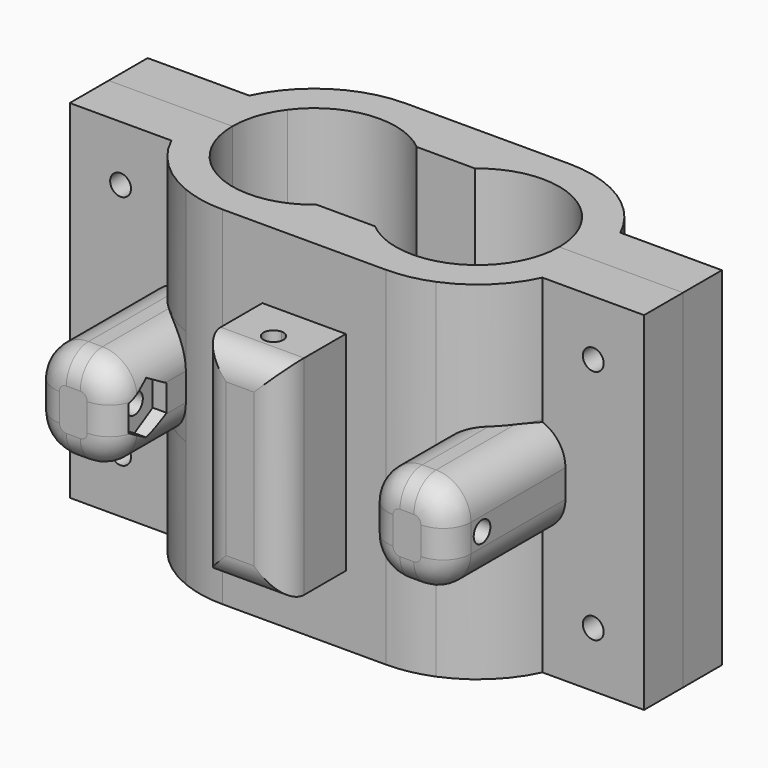
from build123d import *

# Parameters (mm, degrees)
F0_W           = 5.8084472025
F0_H           = 7
F0_W_2         = 1.5
F1_DEPTH       = 50
F2_DEPTH       = 50
F10_START      = -4
F10_DEPTH      = 21
F13_START      = 18
F13_DEPTH      = 14
F11_R          = 1.5
F14_DEPTH      = 35
F14_DEPTH_BACK = 35
F15_R          = 4
F16_START      = 10
F16_DEPTH      = 30
F17_R          = 4
F18_T2_ANGLE   = 90
F18_T4_ANGLE   = 90
F18_T6_ANGLE   = 90
F18_T8_ANGLE   = 90
F18_T10_ANGLE  = 90
F18_T12_ANGLE  = 90
F18_T14_ANGLE  = 90
F18_T16_ANGLE  = 90
F18_T20_DEPTH  = 21
F18_S21_R      = 16.5
F18_T22_DEPTH  = 13
F18_T26_DEPTH  = 21
F18_S27_R      = 16.5
F18_T28_DEPTH  = 13
F18_T32_DEPTH  = 25.2295219459
F18_S33_R      = 16.5
F18_T34_DEPTH  = 15
F18_T38_DEPTH  = 25.2295219459
F18_S39_R      = 16.5
F18_T40_DEPTH  = 15
F18_T44_DEPTH  = 25.2295219459
F18_S45_R      = 16.5
F18_T46_DEPTH  = 15
F18_T50_DEPTH  = 25.2295219459
F18_S51_R      = 16.5
F18_T52_DEPTH  = 15
F18_T56_DEPTH  = 21
F18_S57_R      = 16.5
F18_T58_DEPTH  = 13
F18_T62_DEPTH  = 21
F18_S63_R      = 16.5
F18_T64_DEPTH  = 13
F19_START      = -10
F19_DEPTH      = 10
F20_START      = 10
F20_DEPTH      = 10


# Not quite as in the source:
# - a fillet or chamfer that OpenCascade refuses, or shapes differently, is made with other operations: its cross-section is extruded or revolved along the edge and cut away or added
# - a feature names something its author has since deleted; it is built from what else it names


with BuildPart() as f1:
    # F0 (on Top) → F1 (new body)
    with BuildSketch(Plane.XY):
        with BuildLine():
            Line((-26.6915527975, 7), (-21.1872930441, 7))
            ThreePointArc((-21.1872930441, 7), (-13.1235807588, 11.6694376856), (-4.1960275351, 9))
            Line((-4.1960275351, 9), (4.1960275351, 9))
            ThreePointArc((4.1960275351, 9), (13.1235807588, 11.6694376856), (21.1872930441, 7))
            Line((21.1872930441, 7), (26.6915527975, 7))
            ThreePointArc((26.6915527975, 7), (20.6029656048, 13.9239003156), (11.75, 16.5))
            ThreePointArc((11.75, 16.5), (5.3815186987, 15.2214469061), (0, 11.5839328382))
            ThreePointArc((0, 11.5839328382), (-5.3815186987, 15.2214469061), (-11.75, 16.5))
            ThreePointArc((-11.75, 16.5), (-20.6029656048, 13.9239003156), (-26.6915527975, 7))
        make_face()
        with Locations((38.4042236013, 3.5)):
            Rectangle(F0_W, F0_H)
        with Locations((-38.4042236013, 3.5)):
            Rectangle(F0_W, F0_H)
        with Locations((-34.75, 3.5)):
            Rectangle(F0_W_2, F0_H)
        with Locations((-33.25, 3.5)):
            Rectangle(F0_W_2, F0_H)
        with BuildLine():
            Line((-32.5, 0), (-28.25, 0))
            ThreePointArc((-28.25, 0), (-27.8556763465, 3.585692321), (-26.6915527975, 7))
            Line((-26.6915527975, 7), (-32.5, 7))
            Line((-32.5, 7), (-32.5, 0))
        make_face()
        with Locations((33.25, 3.5)):
            Rectangle(F0_W_2, F0_H)
        with BuildLine():
            ThreePointArc((26.6915527975, 7), (27.8556763465, 3.585692321), (28.25, 0))
            Line((28.25, 0), (32.5, 0))
            Line((32.5, 0), (32.5, 7))
            Line((32.5, 7), (26.6915527975, 7))
        make_face()
        with Locations((34.75, 3.5)):
            Rectangle(F0_W_2, F0_H)
        with BuildLine():
            Line((-28.25, 0), (-23.5, 0))
            ThreePointArc((-23.5, 0), (-22.9068520038, 3.686075605), (-21.1872930441, 7))
            Line((-21.1872930441, 7), (-26.6915527975, 7))
            ThreePointArc((-26.6915527975, 7), (-27.8556763465, 3.585692321), (-28.25, 0))
        make_face()
        with BuildLine():
            ThreePointArc((21.1872930441, 7), (22.9068520038, 3.686075605), (23.5, 0))
            Line((23.5, 0), (28.25, 0))
            ThreePointArc((28.25, 0), (27.8556763465, 3.585692321), (26.6915527975, 7))
            Line((26.6915527975, 7), (21.1872930441, 7))
        make_face()
        with BuildLine():
            Line((11.75, 16.5), (-11.75, 16.5))
            ThreePointArc((-11.75, 16.5), (-5.3815186987, 15.2214469061), (0, 11.5839328382))
            ThreePointArc((0, 11.5839328382), (5.3815186987, 15.2214469061), (11.75, 16.5))
        make_face()
    extrude(amount=F1_DEPTH)


with BuildPart() as f2:
    # F0 (on Top) → F2 (new body)
    with BuildSketch(Plane.XY):
        with Locations((-38.4042236013, -3.5)):
            Rectangle(F0_W, F0_H)
        with Locations((-34.75, -3.5)):
            Rectangle(F0_W_2, F0_H)
        with Locations((-33.25, -3.5)):
            Rectangle(F0_W_2, F0_H)
        with BuildLine():
            ThreePointArc((-26.6915527975, -7), (-27.8556763465, -3.585692321), (-28.25, 0))
            Line((-28.25, 0), (-32.5, 0))
            Line((-32.5, 0), (-32.5, -7))
            Line((-32.5, -7), (-30, -7))
            Line((-30, -7), (-26.6915527975, -7))
        make_face()
        with BuildLine():
            Line((4.1960275351, -9), (-4.1960275351, -9))
            ThreePointArc((-4.1960275351, -9), (-16.7150439846, -10.649452485), (-23.5, 0))
            Line((-23.5, 0), (-28.25, 0))
            ThreePointArc((-28.25, 0), (-27.8556763465, -3.585692321), (-26.6915527975, -7))
            ThreePointArc((-26.6915527975, -7), (-23.1241232323, -11.9532138229), (-18, -15.2704780541))
            ThreePointArc((-18, -15.2704780541), (-14.9348949832, -16.1897017868), (-11.75, -16.5))
            ThreePointArc((-11.75, -16.5), (-5.3815186987, -15.2214469061), (0, -11.5839328382))
            ThreePointArc((0, -11.5839328382), (5.3815186987, -15.2214469061), (11.75, -16.5))
            ThreePointArc((11.75, -16.5), (14.9348949832, -16.1897017868), (18, -15.2704780541))
            ThreePointArc((18, -15.2704780541), (23.1241232323, -11.9532138229), (26.6915527975, -7))
            ThreePointArc((26.6915527975, -7), (27.8556763465, -3.585692321), (28.25, 0))
            Line((28.25, 0), (23.5, 0))
            ThreePointArc((23.5, 0), (16.7150439846, -10.649452485), (4.1960275351, -9))
        make_face()
        with BuildLine():
            Line((32.5, 0), (28.25, 0))
            ThreePointArc((28.25, 0), (27.8556763465, -3.585692321), (26.6915527975, -7))
            Line((26.6915527975, -7), (30, -7))
            Line((30, -7), (32.5, -7))
            Line((32.5, -7), (32.5, 0))
        make_face()
        with Locations((33.25, -3.5)):
            Rectangle(F0_W_2, F0_H)
        with Locations((34.75, -3.5)):
            Rectangle(F0_W_2, F0_H)
        with Locations((38.4042236013, -3.5)):
            Rectangle(F0_W, F0_H)
        with BuildLine():
            ThreePointArc((0, -11.5839328382), (-5.3815186987, -15.2214469061), (-11.75, -16.5))
            Line((-11.75, -16.5), (-6, -16.5))
            Line((-6, -16.5), (0, -16.5))
            Line((0, -16.5), (6, -16.5))
            Line((6, -16.5), (11.75, -16.5))
            ThreePointArc((11.75, -16.5), (5.3815186987, -15.2214469061), (0, -11.5839328382))
        make_face()
    extrude(amount=F2_DEPTH)


with BuildPart() as f3:
    # F0 (on Top) → F3 (revolve)
    with BuildSketch(Plane.XY):
        with Locations((-34.75, 3.5)):
            Rectangle(F0_W_2, F0_H)
        with Locations((-34.75, -3.5)):
            Rectangle(F0_W_2, F0_H)
    revolve(axis=Axis((-34, 3.5, 0), (0, -1, 0)))


with BuildPart() as f4:
    # F0 (on Top) → F4 (revolve)
    with BuildSketch(Plane.XY):
        with Locations((34.75, 3.5)):
            Rectangle(F0_W_2, F0_H)
        with Locations((34.75, -3.5)):
            Rectangle(F0_W_2, F0_H)
    revolve(axis=Axis((34, 3.5, 0), (0, -1, 0)))


with BuildPart() as f5:
    # F0 (on Top) → F5 (revolve)
    with BuildSketch(Plane.XY):
        with Locations((34.75, 3.5)):
            Rectangle(F0_W_2, F0_H)
        with Locations((34.75, -3.5)):
            Rectangle(F0_W_2, F0_H)
    revolve(axis=Axis((34, 3.5, 0), (0, -1, 0)))


with BuildPart() as f6:
    # F0 (on Top) → F6 (revolve)
    with BuildSketch(Plane.XY):
        with Locations((-33.25, 3.5)):
            Rectangle(F0_W_2, F0_H)
        with Locations((-33.25, -3.5)):
            Rectangle(F0_W_2, F0_H)
    revolve(axis=Axis((-34, 3.5, 0), (0, -1, 0)))


with BuildPart() as f3_1:
    # F7: moved
    add(f3.part.moved(Location((0, 0, 42))))


with BuildPart() as f4_1:
    # F7: moved
    add(f4.part.moved(Location((0, 0, 42))))


with BuildPart() as f6_1:
    # F8: moved
    add(f6.part.moved(Location((0, 0, 8))))


with BuildPart() as f5_1:
    # F8: moved
    add(f5.part.moved(Location((0, 0, 8))))


with BuildPart() as f10_tool:
    # F9 (on Front) → F10 (new body)
    with BuildSketch(Plane.XZ.offset(F10_START)):
        Polygon((37.275, 40.1091778684), (37.275, 43.8908221316), (34, 45.7816442632), (30.725, 43.8908221316), (30.725, 40.1091778684), (34, 38.2183557368), align=None)
        Polygon((37.275, 6.1091778684), (37.275, 9.8908221316), (34, 11.7816442632), (30.725, 9.8908221316), (30.725, 6.1091778684), (34, 4.2183557368), align=None)
        Polygon((-30.725, 6.1091778684), (-30.725, 9.8908221316), (-34, 11.7816442632), (-37.275, 9.8908221316), (-37.275, 6.1091778684), (-34, 4.2183557368), align=None)
        Polygon((-30.725, 40.1091778684), (-30.725, 43.8908221316), (-34, 45.7816442632), (-37.275, 43.8908221316), (-37.275, 40.1091778684), (-34, 38.2183557368), align=None)
    extrude(amount=-F10_DEPTH)


with BuildPart() as f1_1:
    add(f1.part)

    # F10: cut by f10_tool
    add(f10_tool.part, mode=Mode.SUBTRACT)


with BuildPart() as f3_2:
    add(f3_1.part)

    # F10: cut by f10_tool
    add(f10_tool.part, mode=Mode.SUBTRACT)


with BuildPart() as f4_2:
    add(f4_1.part)

    # F10: cut by f10_tool
    add(f10_tool.part, mode=Mode.SUBTRACT)


with BuildPart() as f5_2:
    add(f5_1.part)

    # F10: cut by f10_tool
    add(f10_tool.part, mode=Mode.SUBTRACT)


with BuildPart() as f6_2:
    add(f6_1.part)

    # F10: cut by f10_tool
    add(f10_tool.part, mode=Mode.SUBTRACT)


with BuildPart() as f1_2:
    add(f1_1.part)

    # F12: cut F4, F5, F3, F6
    add(f4_2.part, mode=Mode.SUBTRACT)
    add(f5_2.part, mode=Mode.SUBTRACT)
    add(f3_2.part, mode=Mode.SUBTRACT)
    add(f6_2.part, mode=Mode.SUBTRACT)


with BuildPart() as f2_1:
    add(f2.part)

    # F12: cut F4, F5, F3, F6
    add(f4_2.part, mode=Mode.SUBTRACT)
    add(f5_2.part, mode=Mode.SUBTRACT)
    add(f3_2.part, mode=Mode.SUBTRACT)
    add(f6_2.part, mode=Mode.SUBTRACT)

    # F0 (on Top) → F13 (join)
    with BuildSketch(Plane.XY.offset(F13_START)):
        with BuildLine():
            ThreePointArc((-18, -15.2704780541), (-23.1241232323, -11.9532138229), (-26.6915527975, -7))
            Line((-26.6915527975, -7), (-30, -7))
            Line((-30, -7), (-30, -28))
            Line((-30, -28), (-18, -28))
            Line((-18, -28), (-18, -15.2704780541))
        make_face()
        with BuildLine():
            Line((30, -7), (26.6915527975, -7))
            ThreePointArc((26.6915527975, -7), (23.1241232323, -11.9532138229), (18, -15.2704780541))
            Line((18, -15.2704780541), (18, -28))
            Line((18, -28), (30, -28))
            Line((30, -28), (30, -7))
        make_face()
    extrude(amount=F13_DEPTH)

    # F11 (on Right) → F14 (cut, two sides)
    with BuildSketch(Plane.YZ) as f14_sk:
        with Locations((-22, 25)):
            Circle(F11_R)
    extrude(amount=F14_DEPTH, mode=Mode.SUBTRACT)
    extrude(f14_sk.sketch, amount=-F14_DEPTH_BACK, mode=Mode.SUBTRACT)

    # F15
    f15_edges = [f2_1.edges().sort_by_distance(p)[0] for p in [
        (30, -28, 25),
        (24, -28, 18),
        (24, -28, 32),
        (18, -28, 25),
        (-18, -28, 25),
        (-24, -28, 32),
        (-30, -28, 25),
        (-24, -28, 18),
    ]]
    fillet(f15_edges, radius=F15_R)

    # F0 (on Top) → F16 (join)
    with BuildSketch(Plane.XY.offset(F16_START)):
        with BuildLine():
            Line((0, -16.5), (-6, -16.5))
            Line((-6, -16.5), (-6, -28))
            Line((-6, -28), (0, -28))
            Line((0, -28), (0, -23.425))
            ThreePointArc((0, -23.425), (-1.425, -22), (0, -20.575))
            Line((0, -20.575), (0, -16.5))
        make_face()
        with BuildLine():
            Line((6, -28), (6, -16.5))
            Line((6, -16.5), (0, -16.5))
            Line((0, -16.5), (0, -20.575))
            ThreePointArc((0, -20.575), (1.0076271632, -20.9923728368), (1.425, -22))
            ThreePointArc((1.425, -22), (1.0076271632, -23.0076271632), (0, -23.425))
            Line((0, -23.425), (0, -28))
            Line((0, -28), (6, -28))
        make_face()
    extrude(amount=F16_DEPTH)

    # F17
    f17_edges = [f2_1.edges().sort_by_distance(p)[0] for p in [
        (6, -28, 25),
        (0, -28, 40),
        (-6, -28, 25),
        (0, -28, 10),
    ]]
    fillet(f17_edges, radius=F17_R)

    # F18: fillet of radius 5 on 8 edges, made by hand

    # F18_s1 → F18_t2 (revolve, cut)
    with BuildSketch(Plane.XY.offset(23)):
        with BuildLine():
            ThreePointArc((-26, -28), (-28.8284271247, -26.8284271247), (-30, -24))
            Line((-30, -24), (-30, -28))
            Line((-30, -28), (-26, -28))
        make_face()
    revolve(axis=Axis((-25, -28, 23), (0, -1, 0)), revolution_arc=F18_T2_ANGLE, mode=Mode.SUBTRACT)

    # F18_s3 → F18_t4 (revolve, cut)
    with BuildSketch(Plane.YZ.offset(-25)):
        with BuildLine():
            ThreePointArc((-28, 28), (-26.8284271247, 30.8284271247), (-24, 32))
            Line((-24, 32), (-28, 32))
            Line((-28, 32), (-28, 28))
        make_face()
    revolve(axis=Axis((-25, -28, 27), (0, -1, 0)), revolution_arc=F18_T4_ANGLE, mode=Mode.SUBTRACT)

    # F18_s5 → F18_t6 (revolve, cut)
    with BuildSketch(Plane.YZ.offset(-23)):
        with BuildLine():
            ThreePointArc((-28, 22), (-26.8284271247, 19.1715728753), (-24, 18))
            Line((-24, 18), (-28, 18))
            Line((-28, 18), (-28, 22))
        make_face()
    revolve(axis=Axis((-23, -28, 23), (0, -1, 0)), revolution_arc=F18_T6_ANGLE, mode=Mode.SUBTRACT)

    # F18_s7 → F18_t8 (revolve, cut)
    with BuildSketch(Plane.XY.offset(27)):
        with BuildLine():
            ThreePointArc((-22, -28), (-19.1715728753, -26.8284271247), (-18, -24))
            Line((-18, -24), (-18, -28))
            Line((-18, -28), (-22, -28))
        make_face()
    revolve(axis=Axis((-23, -28, 27), (0, -1, 0)), revolution_arc=F18_T8_ANGLE, mode=Mode.SUBTRACT)

    # F18_s9 → F18_t10 (revolve, cut)
    with BuildSketch(Plane.XY.offset(23)):
        with BuildLine():
            ThreePointArc((22, -28), (19.1715728753, -26.8284271247), (18, -24))
            Line((18, -24), (18, -28))
            Line((18, -28), (22, -28))
        make_face()
    revolve(axis=Axis((23, -28, 23), (0, -1, 0)), revolution_arc=F18_T10_ANGLE, mode=Mode.SUBTRACT)

    # F18_s11 → F18_t12 (revolve, cut)
    with BuildSketch(Plane.YZ.offset(23)):
        with BuildLine():
            ThreePointArc((-28, 28), (-26.8284271247, 30.8284271247), (-24, 32))
            Line((-24, 32), (-28, 32))
            Line((-28, 32), (-28, 28))
        make_face()
    revolve(axis=Axis((23, -28, 27), (0, -1, 0)), revolution_arc=F18_T12_ANGLE, mode=Mode.SUBTRACT)

    # F18_s13 → F18_t14 (revolve, cut)
    with BuildSketch(Plane.XY.offset(27)):
        with BuildLine():
            ThreePointArc((26, -28), (28.8284271247, -26.8284271247), (30, -24))
            Line((30, -24), (30, -28))
            Line((30, -28), (26, -28))
        make_face()
    revolve(axis=Axis((25, -28, 27), (0, -1, 0)), revolution_arc=F18_T14_ANGLE, mode=Mode.SUBTRACT)

    # F18_s15 → F18_t16 (revolve, cut)
    with BuildSketch(Plane.YZ.offset(25)):
        with BuildLine():
            ThreePointArc((-28, 22), (-26.8284271247, 19.1715728753), (-24, 18))
            Line((-24, 18), (-28, 18))
            Line((-28, 18), (-28, 22))
        make_face()
    revolve(axis=Axis((25, -28, 23), (0, -1, 0)), revolution_arc=F18_T16_ANGLE, mode=Mode.SUBTRACT)


with BuildPart() as f18_tool18:
    # F18_s19 → F18_t20 (new body)
    with BuildSketch(Plane.XZ.offset(28)):
        with BuildLine():
            ThreePointArc((25, 18), (28.5355339059, 19.4644660941), (30, 23))
            Line((30, 23), (30, 18))
            Line((30, 18), (25, 18))
        make_face()
    extrude(amount=-F18_T20_DEPTH)

    # F18_s21 → F18_t22 (cut, symmetric)
    with BuildSketch(Plane.XY.offset(20.5)):
        with Locations((11.75, 0)):
            Circle(F18_S21_R)
    extrude(amount=F18_T22_DEPTH, both=True, mode=Mode.SUBTRACT)


with BuildPart() as f2_2:
    add(f2_1.part)

    # F18_t17: cut F18_tool18
    add(f18_tool18.part, mode=Mode.SUBTRACT)


with BuildPart() as f18_tool24:
    # F18_s25 → F18_t26 (new body)
    with BuildSketch(Plane.XZ.offset(28)):
        with BuildLine():
            ThreePointArc((25, 32), (28.5355339059, 30.5355339059), (30, 27))
            Line((30, 27), (30, 32))
            Line((30, 32), (25, 32))
        make_face()
    extrude(amount=-F18_T26_DEPTH)

    # F18_s27 → F18_t28 (cut, symmetric)
    with BuildSketch(Plane.XY.offset(29.5)):
        with Locations((11.75, 0)):
            Circle(F18_S27_R)
    extrude(amount=F18_T28_DEPTH, both=True, mode=Mode.SUBTRACT)


with BuildPart() as f2_3:
    add(f2_2.part)

    # F18_t23: cut F18_tool24
    add(f18_tool24.part, mode=Mode.SUBTRACT)


with BuildPart() as f18_tool30:
    # F18_s31 → F18_t32 (new body)
    with BuildSketch(Plane.XZ.offset(2.7704780541)):
        with BuildLine():
            ThreePointArc((18, 27), (19.4644660941, 30.5355339059), (23, 32))
            Line((23, 32), (18, 32))
            Line((18, 32), (18, 27))
        make_face()
    extrude(amount=F18_T32_DEPTH)

    # F18_s33 → F18_t34 (cut, symmetric)
    with BuildSketch(Plane.XY.offset(29.5)):
        with Locations((11.75, 0)):
            Circle(F18_S33_R)
    extrude(amount=F18_T34_DEPTH, both=True, mode=Mode.SUBTRACT)


with BuildPart() as f2_4:
    add(f2_3.part)

    # F18_t29: cut F18_tool30
    add(f18_tool30.part, mode=Mode.SUBTRACT)


with BuildPart() as f18_tool36:
    # F18_s37 → F18_t38 (new body)
    with BuildSketch(Plane.XZ.offset(2.7704780541)):
        with BuildLine():
            ThreePointArc((23, 18), (19.4644660941, 19.4644660941), (18, 23))
            Line((18, 23), (18, 18))
            Line((18, 18), (23, 18))
        make_face()
    extrude(amount=F18_T38_DEPTH)

    # F18_s39 → F18_t40 (cut, symmetric)
    with BuildSketch(Plane.XY.offset(20.5)):
        with Locations((11.75, 0)):
            Circle(F18_S39_R)
    extrude(amount=F18_T40_DEPTH, both=True, mode=Mode.SUBTRACT)


with BuildPart() as f2_5:
    add(f2_4.part)

    # F18_t35: cut F18_tool36
    add(f18_tool36.part, mode=Mode.SUBTRACT)


with BuildPart() as f18_tool42:
    # F18_s43 → F18_t44 (new body)
    with BuildSketch(Plane.XZ.offset(28)):
        with BuildLine():
            ThreePointArc((-23, 32), (-19.4644660941, 30.5355339059), (-18, 27))
            Line((-18, 27), (-18, 32))
            Line((-18, 32), (-23, 32))
        make_face()
    extrude(amount=-F18_T44_DEPTH)

    # F18_s45 → F18_t46 (cut, symmetric)
    with BuildSketch(Plane.XY.offset(29.5)):
        with Locations((-11.75, 0)):
            Circle(F18_S45_R)
    extrude(amount=F18_T46_DEPTH, both=True, mode=Mode.SUBTRACT)


with BuildPart() as f2_6:
    add(f2_5.part)

    # F18_t41: cut F18_tool42
    add(f18_tool42.part, mode=Mode.SUBTRACT)


with BuildPart() as f18_tool48:
    # F18_s49 → F18_t50 (new body)
    with BuildSketch(Plane.XZ.offset(28)):
        with BuildLine():
            ThreePointArc((-18, 23), (-19.4644660941, 19.4644660941), (-23, 18))
            Line((-23, 18), (-18, 18))
            Line((-18, 18), (-18, 23))
        make_face()
    extrude(amount=-F18_T50_DEPTH)

    # F18_s51 → F18_t52 (cut, symmetric)
    with BuildSketch(Plane.XY.offset(20.5)):
        with Locations((-11.75, 0)):
            Circle(F18_S51_R)
    extrude(amount=F18_T52_DEPTH, both=True, mode=Mode.SUBTRACT)


with BuildPart() as f2_7:
    add(f2_6.part)

    # F18_t47: cut F18_tool48
    add(f18_tool48.part, mode=Mode.SUBTRACT)


with BuildPart() as f18_tool54:
    # F18_s55 → F18_t56 (new body)
    with BuildSketch(Plane.XZ.offset(7)):
        with BuildLine():
            ThreePointArc((-25, 32), (-28.5355339059, 30.5355339059), (-30, 27))
            Line((-30, 27), (-30, 32))
            Line((-30, 32), (-25, 32))
        make_face()
    extrude(amount=F18_T56_DEPTH)

    # F18_s57 → F18_t58 (cut, symmetric)
    with BuildSketch(Plane.XY.offset(29.5)):
        with Locations((-11.75, 0)):
            Circle(F18_S57_R)
    extrude(amount=F18_T58_DEPTH, both=True, mode=Mode.SUBTRACT)


with BuildPart() as f2_8:
    add(f2_7.part)

    # F18_t53: cut F18_tool54
    add(f18_tool54.part, mode=Mode.SUBTRACT)


with BuildPart() as f18_tool60:
    # F18_s61 → F18_t62 (new body)
    with BuildSketch(Plane.XZ.offset(7)):
        with BuildLine():
            ThreePointArc((-25, 18), (-28.5355339059, 19.4644660941), (-30, 23))
            Line((-30, 23), (-30, 18))
            Line((-30, 18), (-25, 18))
        make_face()
    extrude(amount=F18_T62_DEPTH)

    # F18_s63 → F18_t64 (cut, symmetric)
    with BuildSketch(Plane.XY.offset(20.5)):
        with Locations((-11.75, 0)):
            Circle(F18_S63_R)
    extrude(amount=F18_T64_DEPTH, both=True, mode=Mode.SUBTRACT)


with BuildPart() as f2_9:
    add(f2_8.part)

    # F18_t59: cut F18_tool60
    add(f18_tool60.part, mode=Mode.SUBTRACT)

    # F11 (on Right) → F19 (cut)
    with BuildSketch(Plane.YZ.offset(F19_START)):
        Polygon((-18.725, 23.1091778684), (-18.725, 26.8908221316), (-22, 28.7816442632), (-25.275, 26.8908221316), (-25.275, 23.1091778684), (-22, 21.2183557368), align=None)
        with Locations((-22, 25)):
            Circle(F11_R, mode=Mode.SUBTRACT)
    extrude(amount=-F19_DEPTH, mode=Mode.SUBTRACT)

    # F11 (on Right) → F20 (cut)
    with BuildSketch(Plane.YZ.offset(F20_START)):
        Polygon((-18.725, 23.1091778684), (-18.725, 26.8908221316), (-22, 28.7816442632), (-25.275, 26.8908221316), (-25.275, 23.1091778684), (-22, 21.2183557368), align=None)
        with Locations((-22, 25)):
            Circle(F11_R, mode=Mode.SUBTRACT)
    extrude(amount=F20_DEPTH, mode=Mode.SUBTRACT)


solid = Compound([f1_2.part, f2_9.part])
